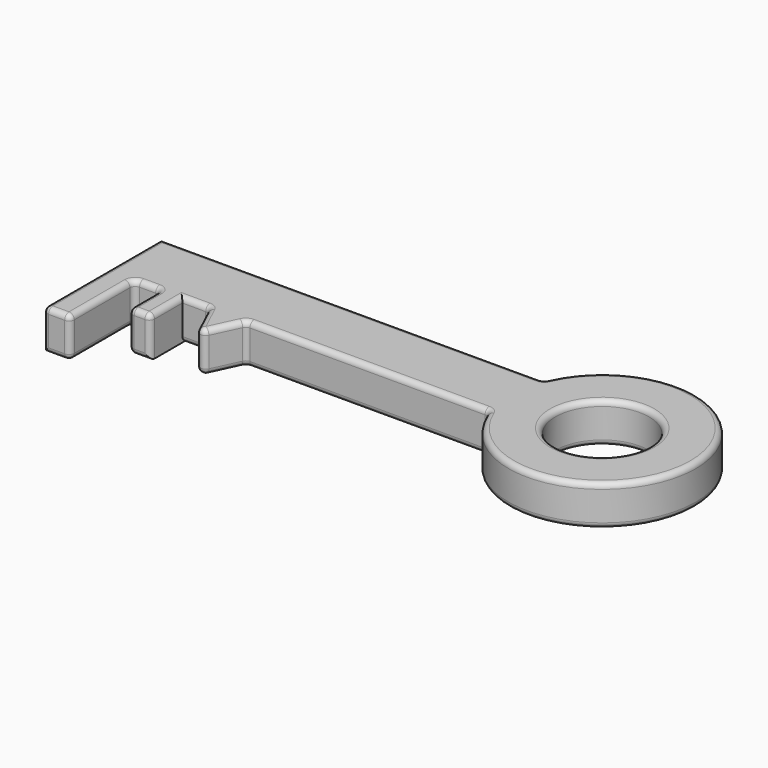
from build123d import *

# Parameters (mm, degrees)
F0_R     = 17.5
F0_W     = 8
F0_H     = 15
F0_W_2   = 10
F0_H_2   = 30
F1_DEPTH = 15
F2_R     = 2


with BuildPart() as f1:
    # F0 (on Top) → F1 (new body)
    with BuildSketch(Plane.XY):
        with BuildLine():
            ThreePointArc((67.9675509022, 0), (135.8918507742, 11.1645103967), (68.4608784178, 25))
            Line((68.4608784178, 25), (-74.5851349286, 25))
            Line((-74.5851349286, 25), (-74.5851349286, 0))
            Line((-74.5851349286, 0), (-64.5851349286, 0))
            Line((-64.5851349286, 0), (-54.5851349286, 0))
            Line((-54.5851349286, 0), (-46.5851349286, 0))
            Line((-46.5851349286, 0), (-36.5851349286, 0))
            Line((-36.5851349286, 0), (-22.5848765024, 0))
            Line((-22.5848765024, 0), (67.9675509022, 0))
        make_face()
        with Locations((100.8986632018, 11.8550344882)):
            Circle(F0_R, mode=Mode.SUBTRACT)
        Polygon((-29.5850057155, -15), (-22.5848765024, 0), (-36.5851349286, 0), align=None)
        with Locations((-50.5851349286, -7.5)):
            Rectangle(F0_W, F0_H)
        with Locations((-69.5851349286, -15)):
            Rectangle(F0_W_2, F0_H_2)
    extrude(amount=F1_DEPTH)

    # F2
    f2_edges = [f1.edges().sort_by_distance(p)[0] for p in [
        (-3.062128, 25, 15),
        (135.891851, 11.16451, 15),
        (-26.084941, -7.5, 15),
        (-46.585135, -7.5, 15),
        (-74.585135, -2.5, 15),
        (-69.585135, -30, 15),
        (-64.585135, -15, 15),
        (-59.585135, 0, 15),
        (-54.585135, -7.5, 15),
        (-50.585135, -15, 15),
        (-41.585135, 0, 15),
        (-33.08507, -7.5, 15),
        (22.691337, 0, 15),
        (83.398663, 11.855034, 15),
        (-46.585135, -15, 7.5),
        (-41.585135, 0, 0),
        (-33.08507, -7.5, 0),
        (22.691337, 0, 0),
        (-74.585135, -30, 7.5),
        (-54.585135, -15, 7.5),
        (-59.585135, 0, 0),
        (83.398663, 11.855034, 0),
        (-3.062128, 25, 0),
        (-26.084941, -7.5, 0),
        (-50.585135, -15, 0),
        (-69.585135, -30, 0),
        (135.891851, 11.16451, 0),
        (-29.585006, -15, 7.5),
        (-22.584877, 0, 7.5),
        (-64.585135, -30, 7.5),
        (-64.585135, 0, 7.5),
        (-64.585135, -15, 0),
        (-36.585135, 0, 7.5),
        (-54.585135, 0, 7.5),
        (68.460878, 25, 7.5),
        (67.967551, 0, 7.5),
        (-54.585135, -7.5, 0),
    ]]
    fillet(f2_edges, radius=F2_R)


solid = f1.part
